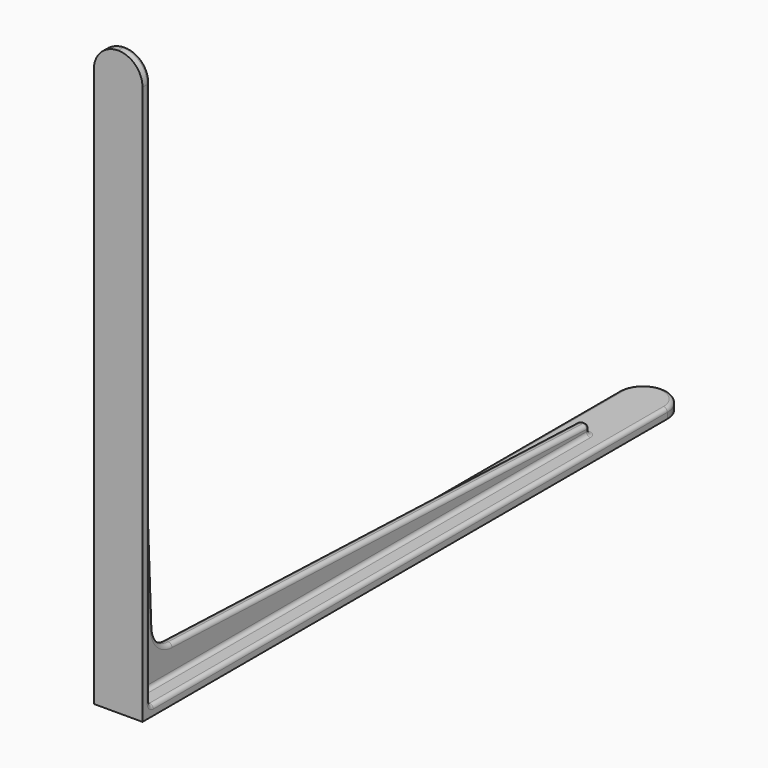
from build123d import *

# Parameters (mm, degrees)
F1_DEPTH = 25
F4_DEPTH = 5
F5_R     = 12.49999
F6_R     = 2


# Not quite as in the source:
# - a fillet or chamfer is up to 0.001 mm smaller than in the source, because OpenCascade refuses the exact size


with BuildPart() as f1:
    # F0 (on Right) → F1 (new body)
    with BuildSketch(Plane.YZ):
        Polygon((0, 300), (0, 0), (350, 0), (350, 5), (5, 5), (5, 300), align=None)
    extrude(amount=-F1_DEPTH)

    # F3 (on offset) → F4 (join)
    with BuildSketch(Plane.YZ.offset(-10)):
        Polygon((10, 250), (5, 250), (5, 5), (300, 5), (300, 10), (20, 20), align=None)
    extrude(amount=-F4_DEPTH)

    # F5 (radius 12.5 in the source; OpenCascade refuses exactly that, so slightly less here)
    f5_edges = [f1.edges().sort_by_distance(p)[0] for p in [
        (0, 2.5, 300),
        (-25, 2.5, 300),
        (-25, 350, 2.5),
        (0, 350, 2.5),
        (-12.5, 20, 20),
    ]]
    fillet(f5_edges, radius=F5_R)

    # F6
    f6_edges = [f1.edges().sort_by_distance(p)[0] for p in [
        (0, 5, 146.250005),
        (-3.661162, 5, 296.338838),
        (-5, 5, 5),
        (-12.5, 5, 300),
        (-10, 5, 127.5),
        (-21.338838, 5, 296.338838),
        (-12.5, 5, 250),
        (-25, 5, 146.250005),
        (-15, 5, 127.5),
        (-20, 5, 5),
        (-10, 14.749198, 140.768451),
        (-12.5, 19.498396, 31.536902),
        (-12.5, 10, 250),
        (-15, 14.749198, 140.768451),
        (-15, 165.770222, 14.793921),
        (-15, 23.182084, 23.206847),
        (-15, 300, 7.5),
        (-15, 152.5, 5),
        (-15, 7.5, 250),
        (-10, 165.770222, 14.793921),
        (-10, 23.182084, 23.206847),
        (-10, 300, 7.5),
        (-10, 152.5, 5),
        (-10, 7.5, 250),
        (0, 171.250005, 5),
        (-3.661162, 346.338838, 5),
        (-12.5, 350, 5),
        (-21.338838, 346.338838, 5),
        (-12.5, 300, 5),
        (-25, 171.250005, 5),
        (-12.5, 300, 10),
    ]]
    fillet(f6_edges, radius=F6_R)


solid = f1.part
